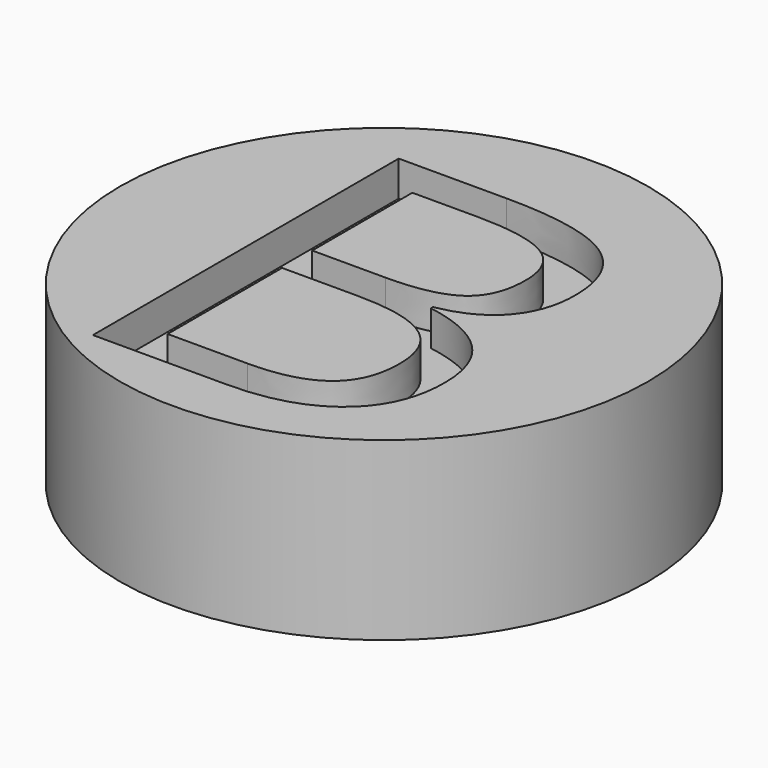
from build123d import *

# Parameters (mm, degrees)
F0_R         = 19.05
F1_DEPTH     = 12.7
F3_START     = 10.16
F2_TEXT_SIZE = 38.6220004752
F3_DEPTH     = 2.54


# Not quite as in the source:
# - Text() gives the source's letters only with a copy of the font that has no kerning and outlines rounded to 1/6400 em; it was checked with that copy


with BuildPart() as f1:
    # F0 (on Top) → F1 (new body)
    with BuildSketch(Plane.XY):
        Circle(F0_R)
    extrude(amount=F1_DEPTH)

    # F2 (on Top) → F3 (cut)
    with BuildSketch(Plane.XY.offset(F3_START)):
        with Locations((-12.7, -15.1078403421)):
            Text('B', F2_TEXT_SIZE, font='Open Sans', text_align=(TextAlign.LEFT, TextAlign.BOTTOM))
    extrude(amount=F3_DEPTH, mode=Mode.SUBTRACT)


solid = f1.part
